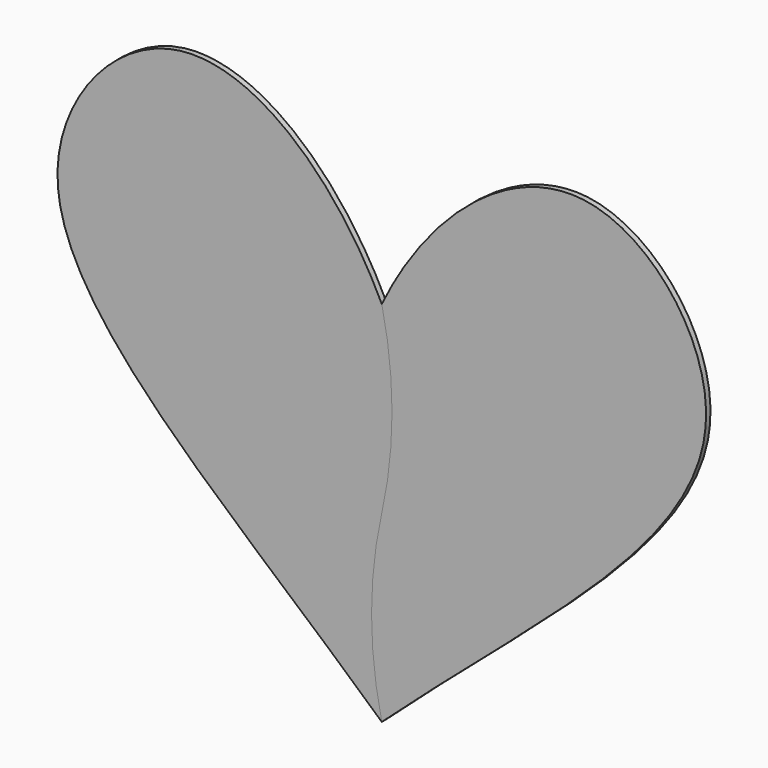
from build123d import *

# Parameters (mm, degrees)
F1_DEPTH = 3
F2_DEPTH = 3


# Not quite as in the source:
# - a feature names something its author has since deleted; it is built from what else it names


with BuildPart() as f1:
    # F0 (on Front) → F1 (new body)
    with BuildSketch(Plane.XZ):
        with BuildLine():
            Line((0, 100), (0, 0))
            add(Edge.make_bspline(
                [(0, 0), (82.3394819819, 75.4575862184), (228.7437395074, 176.365648432), (110.9191157227, 325.2390189646), (25.9574372763, 253.8398247218), (0, 200)],
                knots=[0, 0, 0, 0, 0.4236671268, 0.6921367272, 1, 1, 1, 1], degree=3))
            ThreePointArc((0, 200), (5.5646149333, 150), (0, 100))
        make_face()
        with BuildLine():
            ThreePointArc((0, 100), (-5.578394677, 50), (0, 0))
            Line((0, 0), (0, 100))
        make_face()
    extrude(amount=F1_DEPTH)


with BuildPart() as f2:
    # F0 (on Front) → F2 (new body)
    with BuildSketch(Plane.XZ):
        with BuildLine():
            ThreePointArc((0, 100), (5.5646149333, 150), (0, 200))
            Line((0, 200), (0, 100))
        make_face()
        with BuildLine():
            add(Edge.make_bspline(
                [(0, 0), (-82.3394819819, 75.4575862184), (-228.7437395074, 176.365648432), (-110.9191157227, 325.2390189646), (-25.9574372763, 253.8398247218), (0, 200)],
                knots=[0, 0, 0, 0, 0.4236671268, 0.6921367272, 1, 1, 1, 1], degree=3))
            ThreePointArc((0, 0), (-5.578394677, 50), (0, 100))
            Line((0, 100), (0, 200))
        make_face()
    extrude(amount=F2_DEPTH)


solid = Compound([f1.part, f2.part])
